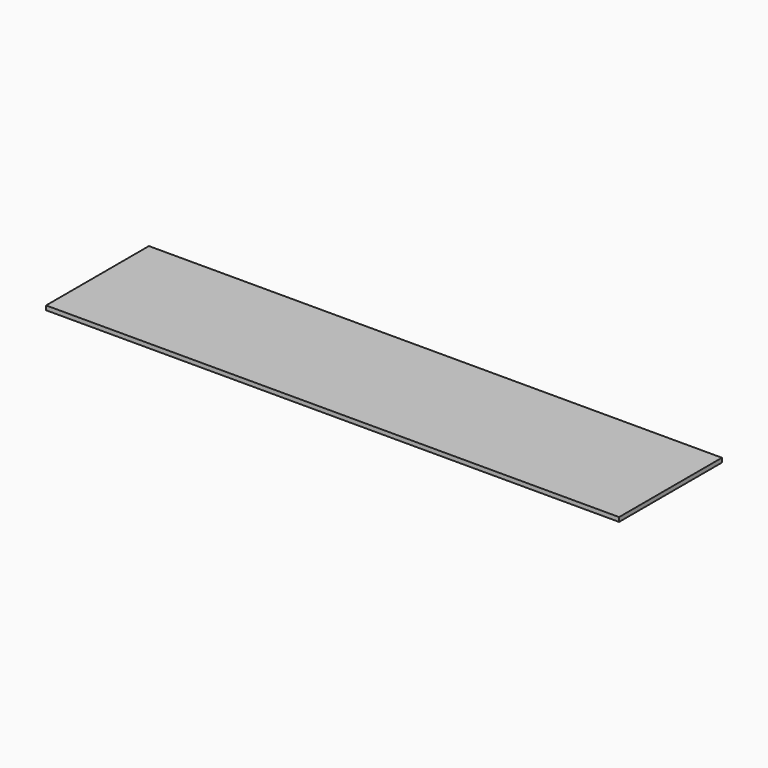
from build123d import *

# Parameters (mm, degrees)
F0_W     = 339.725
F0_H     = 76.2
F1_DEPTH = 2.54


# Not quite as in the source:
# - a feature names something its author has since deleted; it is built from what else it names


with BuildPart() as f1:
    # F0 (on Top) → F1 (new body)
    with BuildSketch(Plane.XY):
        with Locations((169.8625, -38.1)):
            Rectangle(F0_W, F0_H)
    extrude(amount=F1_DEPTH)


solid = f1.part
